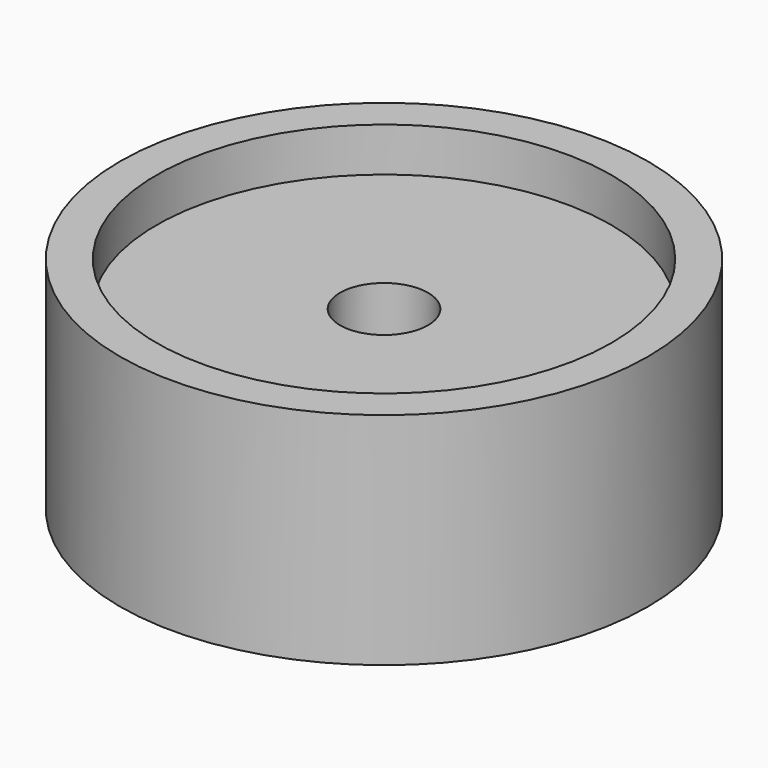
from build123d import *

# Parameters (mm, degrees)
F0_R     = 15.5
F0_R_2   = 12.5
F0_R_3   = 3
F1_DEPTH = 12
F0_R_4   = 18
F2_DEPTH = 15


# Not quite as in the source:
# - a feature names something its author has since deleted; it is built from what else it names


with BuildPart() as f1:
    # F0 (on Top) → F1 (new body)
    with BuildSketch(Plane.XY):
        Circle(F0_R)
        Circle(F0_R_2, mode=Mode.SUBTRACT)
        Circle(F0_R_2)
        Circle(F0_R_3, mode=Mode.SUBTRACT)
    extrude(amount=F1_DEPTH)

    # F0 (on Top) → F2 (join)
    with BuildSketch(Plane.XY):
        Circle(F0_R_4)
        Circle(F0_R, mode=Mode.SUBTRACT)
    extrude(amount=F2_DEPTH)


solid = f1.part
